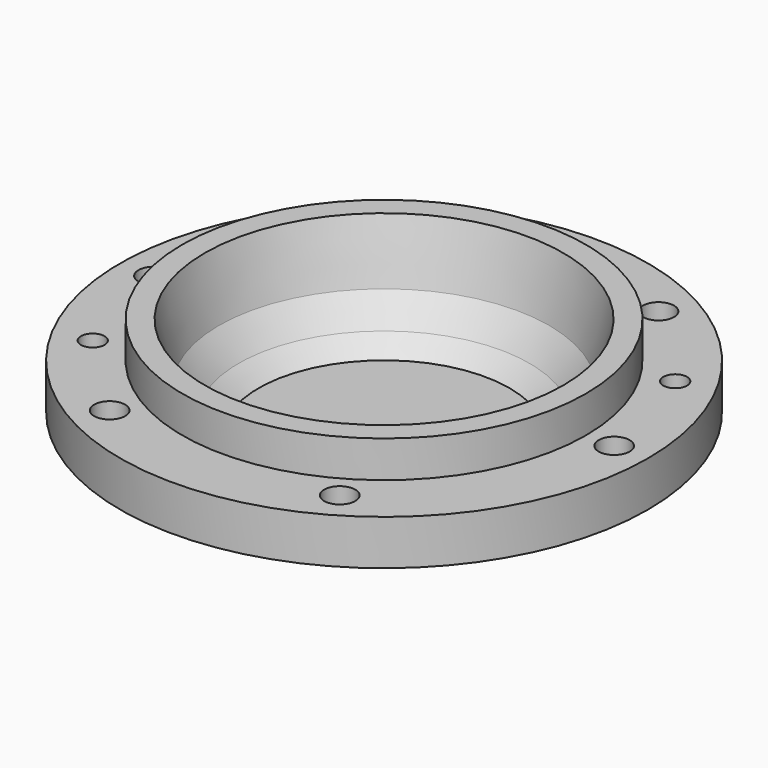
from build123d import *

# Parameters (mm, degrees)
F0_R     = 93.5
F0_R_2   = 5.5
F0_R_3   = 4.2
F0_R_4   = 71.5
F1_DEPTH = 16
F0_R_5   = 67.5
F0_R_6   = 40
F2_DEPTH = 29
F3_DEPTH = 16
F4_R     = 15.99999
F0_R_7   = 5.6
F5_DEPTH = 15


# Not quite as in the source:
# - a fillet or chamfer is up to 0.001 mm smaller than in the source, because OpenCascade refuses the exact size


with BuildPart() as f1:
    # F0 (on Top) → F1 (new body)
    with BuildSketch(Plane.XY):
        Circle(F0_R)
        with Locations((-40.75, -70.5810704084)):
            Circle(F0_R_2, mode=Mode.SUBTRACT)
        with Locations((-70.5181, -40.85)):
            Circle(F0_R_3, mode=Mode.SUBTRACT)
        with Locations((-81.5, 0)):
            Circle(F0_R_2, mode=Mode.SUBTRACT)
        Circle(F0_R_4, mode=Mode.SUBTRACT)
        with Locations((40.75, -70.5810704084)):
            Circle(F0_R_2, mode=Mode.SUBTRACT)
        with Locations((81.5, 0)):
            Circle(F0_R_2, mode=Mode.SUBTRACT)
        with Locations((-40.75, 70.5810704084)):
            Circle(F0_R_2, mode=Mode.SUBTRACT)
        with Locations((70.5181, 40.75)):
            Circle(F0_R_3, mode=Mode.SUBTRACT)
        with Locations((40.75, 70.5810704084)):
            Circle(F0_R_2, mode=Mode.SUBTRACT)
    extrude(amount=F1_DEPTH)

    # F0 (on Top) → F2 (join)
    with BuildSketch(Plane.XY):
        Circle(F0_R_4)
        Circle(F0_R_5, mode=Mode.SUBTRACT)
        Circle(F0_R_5)
        Circle(F0_R_6, mode=Mode.SUBTRACT)
    extrude(amount=F2_DEPTH)

    # F0 (on Top) → F3 (join)
    with BuildSketch(Plane.XY):
        Circle(F0_R_5)
        Circle(F0_R_6, mode=Mode.SUBTRACT)
    extrude(amount=-F3_DEPTH)

    # F4 (radius 16 in the source; OpenCascade refuses exactly that, so slightly less here)
    f4_edges = [f1.edges().sort_by_distance(p)[0] for p in [
        (-67.5, 0, -16),
    ]]
    fillet(f4_edges, radius=F4_R)

    # F0 (on Top) → F5 (join)
    with BuildSketch(Plane.XY):
        Circle(F0_R_6)
        Circle(F0_R_7, mode=Mode.SUBTRACT)
    extrude(amount=-F5_DEPTH)

    # F6 (on Front) → F7 (revolve, cut)
    with BuildSketch(Plane.XZ):
        Polygon((0, 29.0000022426), (0, 8.0000022426), (58.5, 8.0000022426), (63.5, 29.0000022426), align=None)
    revolve(axis=Axis((0, 0, 18.5000022426), (0, 0, 1)), mode=Mode.SUBTRACT)

    # F8 (on Front) → F9 (revolve, cut)
    with BuildSketch(Plane.XZ):
        Polygon((44.5, -6.9999977574), (51.4999961092, -1.4999977574), (58.5, 8.0000022426), (0, 8.0000022426), (0, -1.4999977574), (0, -6.9999977574), align=None)
    revolve(axis=Axis((0, 0, 3.2500022426), (0, 0, 1)), mode=Mode.SUBTRACT)


solid = f1.part
